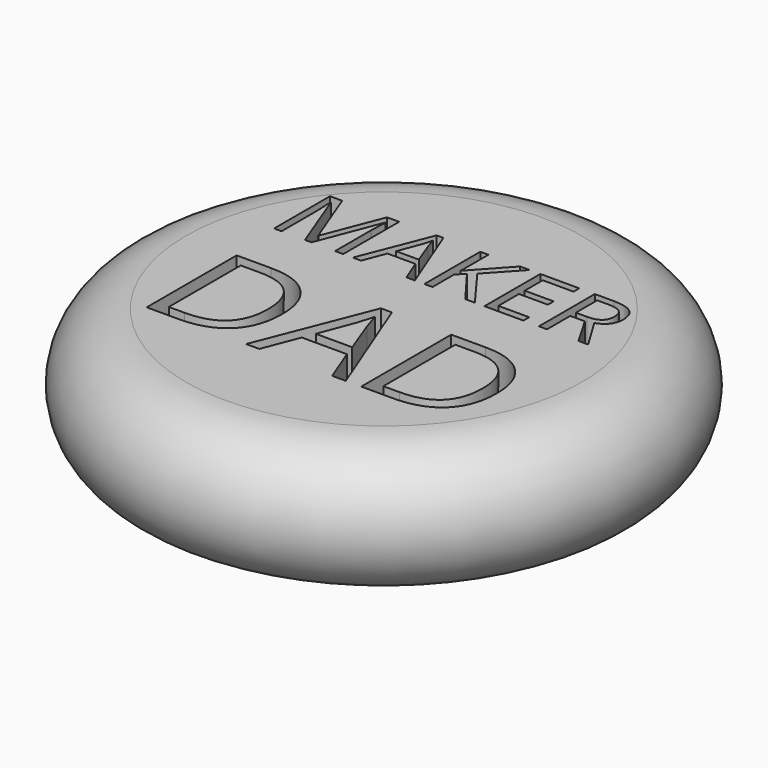
from build123d import *

# Parameters (mm, degrees)
F2_TEXT_SIZE   = 37.6697409278
F2_TEXT_SIZE_2 = 60.6295688498
F3_DEPTH       = 190.5


# Not quite as in the source:
# - Text() gives the source's letters only with a copy of the font that has no kerning and outlines rounded to 1/6400 em; it was checked with that copy


with BuildPart() as f1:
    # F0 (on Front) → F1 (revolve)
    with BuildSketch(Plane.XZ):
        with BuildLine():
            Line((41.4892770014, 39.4531729651), (-34.7107229986, 39.4531729651))
            ThreePointArc((-34.7107229986, 39.4531729651), (-60.1107229986, 14.0531729651), (-34.7107229986, -11.3468270349))
            Line((-34.7107229986, -11.3468270349), (41.4892770014, -11.3468270349))
            Line((41.4892770014, -11.3468270349), (41.4892770014, 39.4531729651))
        make_face()
    revolve(axis=Axis((41.4892770014, 0, 14.0531729651), (0, 0, 1)))

    # F2 (on Top) → F3 (cut, symmetric)
    with BuildSketch(Plane.XY):
        with Locations((-20.6977675494, 20.3120328875)):
            Text('MAKER', F2_TEXT_SIZE, font='Open Sans', text_align=(TextAlign.LEFT, TextAlign.BOTTOM))
        with Locations((-20.790141739, -43.6532895718)):
            Text('DAD', F2_TEXT_SIZE_2, font='Open Sans', text_align=(TextAlign.LEFT, TextAlign.BOTTOM))
    extrude(amount=F3_DEPTH, both=True, mode=Mode.SUBTRACT)


solid = f1.part
